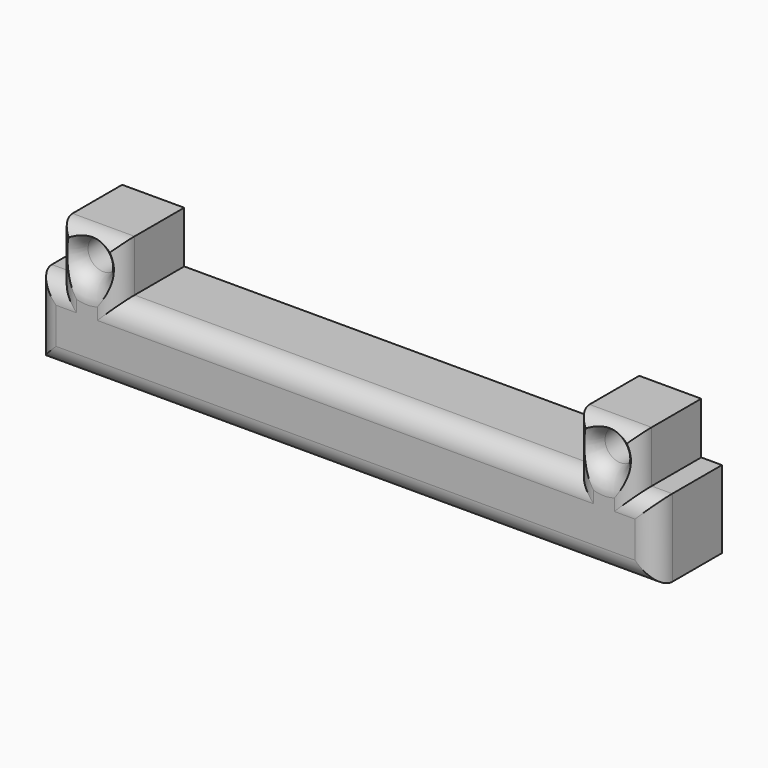
from build123d import *

# Parameters (mm, degrees)
F0_R         = 1.5
F1_DEPTH     = 8
F2_T1_DEPTH  = 17.5
F2_T3_DEPTH  = 70
F2_T5_DEPTH  = 7
F2_T7_DEPTH  = 10
F2_T9_DEPTH  = 16
F2_T11_DEPTH = 44
F2_T13_DEPTH = 16
F2_T15_DEPTH = 7
F2_T25_DEPTH = 12
F2_T29_DEPTH = 15
F2_T36_DEPTH = 15
F2_T40_DEPTH = 49
F2_T47_DEPTH = 49
F2_T51_DEPTH = 15
F2_T58_DEPTH = 15
F2_T62_DEPTH = 12


# Not quite as in the source:
# - a fillet or chamfer that OpenCascade refuses, or shapes differently, is made with other operations: its cross-section is extruded or revolved along the edge and cut away or added


with BuildPart() as f1:
    # F0 (on Front) → F1 (new body)
    with BuildSketch(Plane.XZ):
        Polygon((-55, 7.5), (-55, 0), (5, 0), (5, 7.5), (3, 7.5), (3, 12.5), (-3, 12.5), (-3, 7.5), (-47, 7.5), (-47, 12.5), (-53, 12.5), (-53, 7.5), align=None)
        with Locations((-50, 10)):
            Circle(F0_R, mode=Mode.SUBTRACT)
        with Locations((0, 10)):
            Circle(F0_R, mode=Mode.SUBTRACT)
    extrude(amount=F1_DEPTH)

    # F2: fillet of radius 2 on 14 edges, made by hand

    # F2_s2 → F2_t1 (cut)
    with BuildSketch(Plane.XY.offset(-5)):
        with BuildLine():
            ThreePointArc((-55, -6), (-54.4142135624, -7.4142135624), (-53, -8))
            Line((-53, -8), (-55, -8))
            Line((-55, -8), (-55, -6))
        make_face()
        with BuildLine():
            ThreePointArc((5, -6), (4.4142135624, -7.4142135624), (3, -8))
            Line((3, -8), (5, -8))
            Line((5, -8), (5, -6))
        make_face()
    extrude(amount=F2_T1_DEPTH, mode=Mode.SUBTRACT)

    # F2_s4 → F2_t3 (cut)
    with BuildSketch(Plane.YZ.offset(-60)):
        with BuildLine():
            ThreePointArc((-6, 0), (-7.4142135624, 0.5857864376), (-8, 2))
            Line((-8, 2), (-8, 0))
            Line((-8, 0), (-6, 0))
        make_face()
    extrude(amount=F2_T3_DEPTH, mode=Mode.SUBTRACT)

    # F2_s6 → F2_t5 (cut)
    with BuildSketch(Plane.YZ.offset(3)):
        with BuildLine():
            ThreePointArc((-6, 7.5), (-7.4142135624, 6.9142135624), (-8, 5.5))
            Line((-8, 5.5), (-8, 7.5))
            Line((-8, 7.5), (-6, 7.5))
        make_face()
    extrude(amount=F2_T5_DEPTH, mode=Mode.SUBTRACT)

    # F2_s8 → F2_t7 (cut)
    with BuildSketch(Plane.XY.offset(7.5)):
        with BuildLine():
            ThreePointArc((3, -6), (2.4142135624, -7.4142135624), (1, -8))
            Line((1, -8), (3, -8))
            Line((3, -8), (3, -6))
        make_face()
        with BuildLine():
            ThreePointArc((-3, -6), (-2.4142135624, -7.4142135624), (-1, -8))
            Line((-1, -8), (-3, -8))
            Line((-3, -8), (-3, -6))
        make_face()
        with BuildLine():
            ThreePointArc((-47, -6), (-47.5857864376, -7.4142135624), (-49, -8))
            Line((-49, -8), (-47, -8))
            Line((-47, -8), (-47, -6))
        make_face()
        with BuildLine():
            ThreePointArc((-53, -6), (-52.4142135624, -7.4142135624), (-51, -8))
            Line((-51, -8), (-53, -8))
            Line((-53, -8), (-53, -6))
        make_face()
    extrude(amount=F2_T7_DEPTH, mode=Mode.SUBTRACT)

    # F2_s10 → F2_t9 (cut)
    with BuildSketch(Plane.YZ.offset(-8)):
        with BuildLine():
            ThreePointArc((-6, 12.5), (-7.4142135624, 11.9142135624), (-8, 10.5))
            Line((-8, 10.5), (-8, 12.5))
            Line((-8, 12.5), (-6, 12.5))
        make_face()
    extrude(amount=F2_T9_DEPTH, mode=Mode.SUBTRACT)

    # F2_s12 → F2_t11 (cut)
    with BuildSketch(Plane.YZ.offset(-47)):
        with BuildLine():
            ThreePointArc((-6, 7.5), (-7.4142135624, 6.9142135624), (-8, 5.5))
            Line((-8, 5.5), (-8, 7.5))
            Line((-8, 7.5), (-6, 7.5))
        make_face()
    extrude(amount=F2_T11_DEPTH, mode=Mode.SUBTRACT)

    # F2_s14 → F2_t13 (cut)
    with BuildSketch(Plane.YZ.offset(-58)):
        with BuildLine():
            ThreePointArc((-6, 12.5), (-7.4142135624, 11.9142135624), (-8, 10.5))
            Line((-8, 10.5), (-8, 12.5))
            Line((-8, 12.5), (-6, 12.5))
        make_face()
    extrude(amount=F2_T13_DEPTH, mode=Mode.SUBTRACT)

    # F2_s16 → F2_t15 (cut)
    with BuildSketch(Plane.YZ.offset(-60)):
        with BuildLine():
            ThreePointArc((-6, 7.5), (-7.4142135624, 6.9142135624), (-8, 5.5))
            Line((-8, 5.5), (-8, 7.5))
            Line((-8, 7.5), (-6, 7.5))
        make_face()
    extrude(amount=F2_T15_DEPTH, mode=Mode.SUBTRACT)

    # F2_s17 → F2_t18 (revolve, cut)
    with BuildSketch(Plane.XY.offset(10)):
        with BuildLine():
            ThreePointArc((-48.5, -6), (-47.9142135624, -7.4142135624), (-46.5, -8))
            Line((-46.5, -8), (-48.5, -8))
            Line((-48.5, -8), (-48.5, -6))
        make_face()
    revolve(axis=Axis((-50, -8, 10), (0, -1, 0)), mode=Mode.SUBTRACT)

    # F2_s19 → F2_t20 (revolve, cut)
    with BuildSketch(Plane.XY.offset(10)):
        with BuildLine():
            ThreePointArc((1.5, -6), (2.0857864376, -7.4142135624), (3.5, -8))
            Line((3.5, -8), (1.5, -8))
            Line((1.5, -8), (1.5, -6))
        make_face()
    revolve(axis=Axis((0, -8, 10), (0, -1, 0)), mode=Mode.SUBTRACT)


with BuildPart() as f2_tool23:
    # F2_s24 → F2_t25 (new body)
    with BuildSketch(Plane.YZ.offset(10)):
        with BuildLine():
            ThreePointArc((-6, 7.5), (-7.4142135624, 6.9142135624), (-8, 5.5))
            Line((-8, 5.5), (-8, 7.5))
            Line((-8, 7.5), (-6, 7.5))
        make_face()
    extrude(amount=-F2_T25_DEPTH)

    split(bisect_by=Plane.YZ.offset(3), keep=Keep.BOTTOM)


with BuildPart() as f2_tool27:
    # F2_s28 → F2_t29 (new body)
    with BuildSketch(Plane.XY.offset(2.5)):
        with BuildLine():
            ThreePointArc((3, -6), (2.4142135624, -7.4142135624), (1, -8))
            Line((1, -8), (3, -8))
            Line((3, -8), (3, -6))
        make_face()
    extrude(amount=F2_T29_DEPTH)

    split(bisect_by=Plane.XY.offset(7.5), keep=Keep.BOTTOM)


with BuildPart() as f2_tool23_1:
    add(f2_tool23.part)

    # F2_t31: intersect F2_tool27
    add(f2_tool27.part, mode=Mode.INTERSECT)


with BuildPart() as f1_1:
    add(f1.part)

    # F2_t21: cut F2_tool23
    add(f2_tool23_1.part, mode=Mode.SUBTRACT)


with BuildPart() as f2_tool34:
    # F2_s35 → F2_t36 (new body)
    with BuildSketch(Plane.XY.offset(17.5)):
        with BuildLine():
            ThreePointArc((-3, -6), (-2.4142135624, -7.4142135624), (-1, -8))
            Line((-1, -8), (-3, -8))
            Line((-3, -8), (-3, -6))
        make_face()
    extrude(amount=-F2_T36_DEPTH)

    split(bisect_by=Plane.XY.offset(7.5), keep=Keep.BOTTOM)


with BuildPart() as f2_tool38:
    # F2_s39 → F2_t40 (new body)
    with BuildSketch(Plane.YZ.offset(2)):
        with BuildLine():
            ThreePointArc((-6, 7.5), (-7.4142135624, 6.9142135624), (-8, 5.5))
            Line((-8, 5.5), (-8, 7.5))
            Line((-8, 7.5), (-6, 7.5))
        make_face()
    extrude(amount=-F2_T40_DEPTH)

    split(bisect_by=Plane.YZ.offset(-3), keep=Keep.TOP)


with BuildPart() as f2_tool34_1:
    add(f2_tool34.part)

    # F2_t42: intersect F2_tool38
    add(f2_tool38.part, mode=Mode.INTERSECT)


with BuildPart() as f1_2:
    add(f1_1.part)

    # F2_t32: cut F2_tool34
    add(f2_tool34_1.part, mode=Mode.SUBTRACT)


with BuildPart() as f2_tool45:
    # F2_s46 → F2_t47 (new body)
    with BuildSketch(Plane.YZ.offset(-3)):
        with BuildLine():
            ThreePointArc((-6, 7.5), (-7.4142135624, 6.9142135624), (-8, 5.5))
            Line((-8, 5.5), (-8, 7.5))
            Line((-8, 7.5), (-6, 7.5))
        make_face()
    extrude(amount=-F2_T47_DEPTH)

    split(bisect_by=Plane.YZ.offset(-47), keep=Keep.BOTTOM)


with BuildPart() as f2_tool49:
    # F2_s50 → F2_t51 (new body)
    with BuildSketch(Plane.XY.offset(2.5)):
        with BuildLine():
            ThreePointArc((-47, -6), (-47.5857864376, -7.4142135624), (-49, -8))
            Line((-49, -8), (-47, -8))
            Line((-47, -8), (-47, -6))
        make_face()
    extrude(amount=F2_T51_DEPTH)

    split(bisect_by=Plane.XY.offset(7.5), keep=Keep.BOTTOM)


with BuildPart() as f2_tool45_1:
    add(f2_tool45.part)

    # F2_t53: intersect F2_tool49
    add(f2_tool49.part, mode=Mode.INTERSECT)


with BuildPart() as f1_3:
    add(f1_2.part)

    # F2_t43: cut F2_tool45
    add(f2_tool45_1.part, mode=Mode.SUBTRACT)


with BuildPart() as f2_tool56:
    # F2_s57 → F2_t58 (new body)
    with BuildSketch(Plane.XY.offset(17.5)):
        with BuildLine():
            ThreePointArc((-53, -6), (-52.4142135624, -7.4142135624), (-51, -8))
            Line((-51, -8), (-53, -8))
            Line((-53, -8), (-53, -6))
        make_face()
    extrude(amount=-F2_T58_DEPTH)

    split(bisect_by=Plane.XY.offset(7.5), keep=Keep.BOTTOM)


with BuildPart() as f2_tool60:
    # F2_s61 → F2_t62 (new body)
    with BuildSketch(Plane.YZ.offset(-48)):
        with BuildLine():
            ThreePointArc((-6, 7.5), (-7.4142135624, 6.9142135624), (-8, 5.5))
            Line((-8, 5.5), (-8, 7.5))
            Line((-8, 7.5), (-6, 7.5))
        make_face()
    extrude(amount=-F2_T62_DEPTH)

    split(bisect_by=Plane.YZ.offset(-53), keep=Keep.TOP)


with BuildPart() as f2_tool56_1:
    add(f2_tool56.part)

    # F2_t64: intersect F2_tool60
    add(f2_tool60.part, mode=Mode.INTERSECT)


with BuildPart() as f1_4:
    add(f1_3.part)

    # F2_t54: cut F2_tool56
    add(f2_tool56_1.part, mode=Mode.SUBTRACT)


solid = f1_4.part
